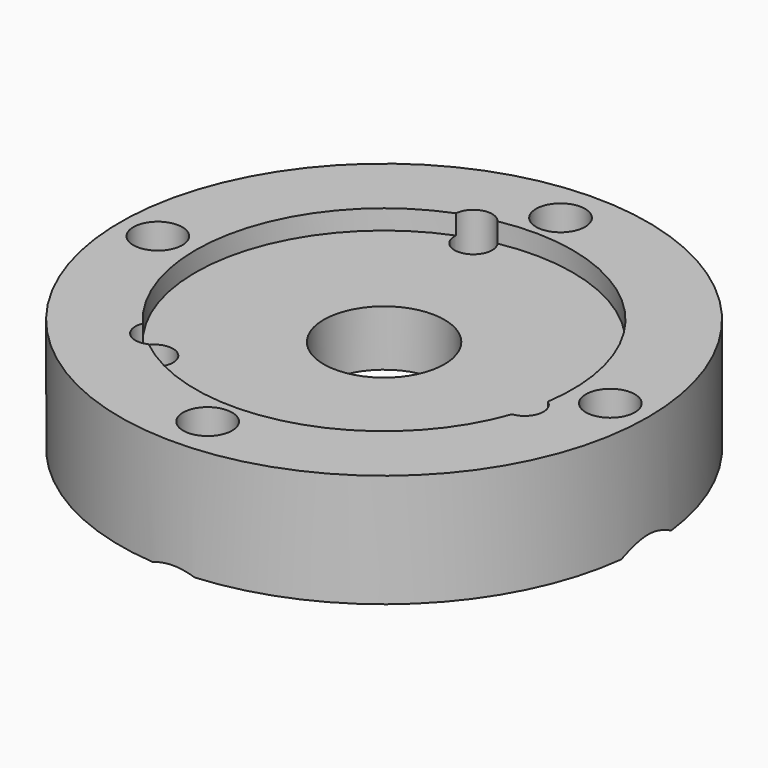
from build123d import *

# Parameters (mm, degrees)
F0_R           = 35
F1_DEPTH       = 15
F2_R           = 25
F3_DEPTH       = 2.6
F4_R           = 18
F5_DEPTH       = 5
F6_D           = 5
F7_D           = 6.5
F7_CSINK_D     = 12.6
F7_CSINK_ANGLE = 90
F8_D           = 16


with BuildPart() as f1:
    # F0 (on Top) → F1 (new body)
    with BuildSketch(Plane.XY):
        Circle(F0_R)
    extrude(amount=F1_DEPTH)

    # F2 (on face) → F3 (cut)
    with BuildSketch(Plane.XY.offset(15)):
        Circle(F2_R)
    extrude(amount=-F3_DEPTH, mode=Mode.SUBTRACT)

    # F4 (on face) → F5 (cut)
    with BuildSketch(Plane(origin=(0, 0, 0), x_dir=(1, 0, 0), z_dir=(0, 0, -1))):
        Circle(F4_R)
    extrude(amount=-F5_DEPTH, mode=Mode.SUBTRACT)

    # F6 (through all)
    with Locations(Plane(origin=(0, 0, 0), x_dir=(1, 0, 0), z_dir=(0, 0, -1))):
        with Locations((-6.6152965396, -23.0702807025), (-16.671800891, 17.2641552081), (23.2870974306, 5.8061254944)):
            Hole(F6_D / 2)

    # F7 (through all)
    with Locations(Plane(origin=(0, 0, 0), x_dir=(1, 0, 0), z_dir=(0, 0, -1))):
        with Locations((30, 0), (-30, 0), (0, -29.25), (0, 29.25)):
            CounterSinkHole(F7_D / 2, F7_CSINK_D / 2, counter_sink_angle=F7_CSINK_ANGLE)

    # F8 (through all)
    with Locations(Plane(origin=(0, 0, 0), x_dir=(1, 0, 0), z_dir=(0, 0, -1))):
        with Locations((0, 0)):
            Hole(F8_D / 2)


solid = f1.part
